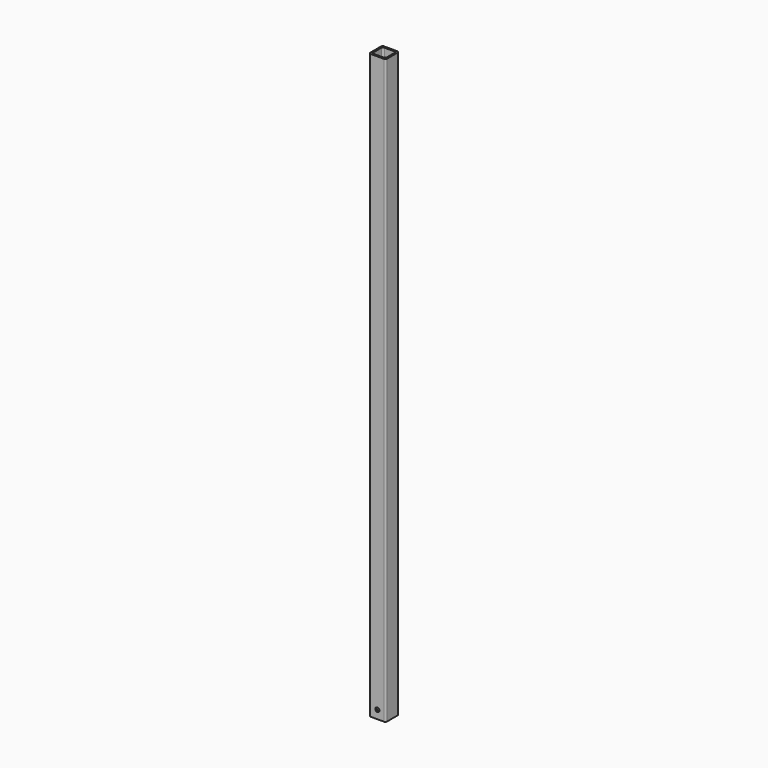
from build123d import *

# Parameters (mm, degrees)
F0_W     = 20
F0_H     = 20
F1_DEPTH = 700
F2_R     = 2
F3_T     = 2
F4_R     = 2
F5_R     = 2.5
F6_DEPTH = 25.2


# Not quite as in the source:
# - a shell that OpenCascade refuses in one call is made with other operations: the cavity is built on its own and cut out


with BuildPart() as f1:
    # F0 (on Top) → F1 (new body)
    with BuildSketch(Plane.XY):
        Rectangle(F0_W, F0_H)
    extrude(amount=F1_DEPTH)

    # F2
    f2_edges = [f1.edges().sort_by_distance(p)[0] for p in [
        (-10, 10, 350),
        (-10, -10, 350),
        (10, -10, 350),
        (10, 10, 350),
    ]]
    fillet(f2_edges, radius=F2_R)

    # F3: shell of thickness 2, made by hand


with BuildPart() as f3_core1:
    # F3_t2: copy of F1
    add(f1.part)

    # the walls: a layer under each face that stays
    f3_faces = [f3_core1.faces().sort_by_distance(p)[0] for p in [
        (0, -10, 350),
        (-10, 0, 350),
        (10, 0, 350),
        (0, 10, 350),
    ]]
    thicken(f3_faces, amount=-F3_T, mode=Mode.SUBTRACT)


with BuildPart() as f1_1:
    add(f1.part)

    # what is left inside the walls is the cavity
    f3_cavity = [f3_core1.part.solids().sort_by_distance(p)[0] for p in [
        (-7.98, 0, 466.666667),
    ]]
    add(f3_cavity, mode=Mode.SUBTRACT)

    # F4
    f4_edges = [f1_1.edges().sort_by_distance(p)[0] for p in [
        (-8, 8, 350),
        (-8, -8, 350),
        (8, -8, 350),
        (8, 8, 350),
    ]]
    fillet(f4_edges, radius=F4_R)

    # F5 (on face) → F6 (cut)
    with BuildSketch(Plane(origin=(0, 10, 0), x_dir=(-1, 0, 0), z_dir=(0, 1, 0))):
        with Locations((0, 10)):
            Circle(F5_R)
    extrude(amount=-F6_DEPTH, mode=Mode.SUBTRACT)


solid = f1_1.part
